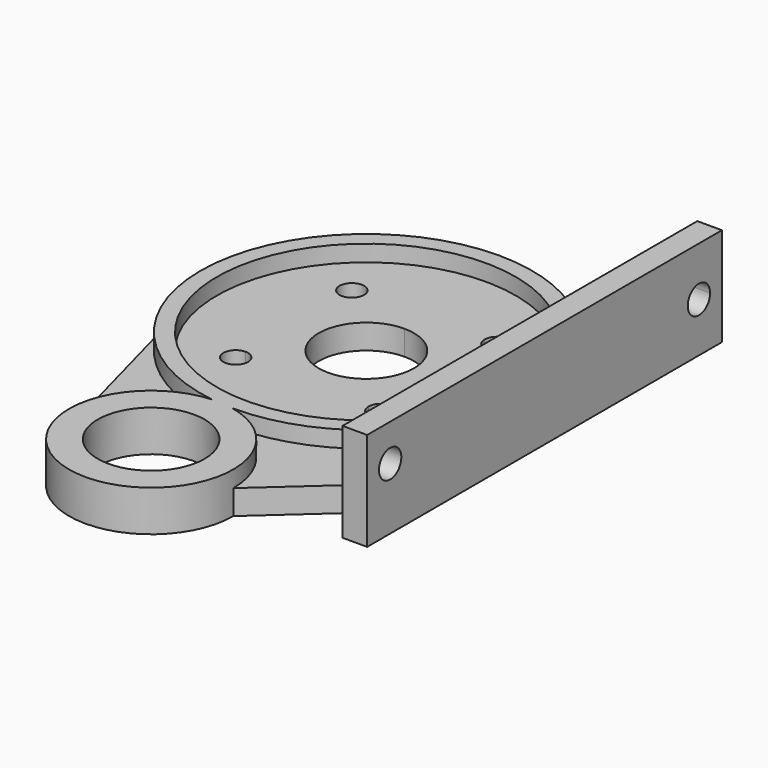
from build123d import *

# Parameters (mm, degrees)
F0_W     = 3
F0_H     = 6.8
F1_DEPTH = 12
F2_DEPTH = 5
F3_DEPTH = 3
F0_R     = 6.5
F4_DEPTH = 5
F5_DEPTH = 3
F7_DEPTH = 25
F8_DEPTH = 25
F9_DEPTH = 3


with BuildPart() as f1:
    # F0 (on Top) → F1 (new body)
    with BuildSketch(Plane.XY):
        with Locations((20.2, 23.6)):
            Rectangle(F0_W, F0_H)
        with BuildLine():
            Line((18.7, 20.2), (18.7, 7.6387171698))
            ThreePointArc((18.7, 7.6387171698), (19.8214530244, 3.8923000912), (20.2, 0))
            Line((20.2, 0), (21.7, 0))
            Line((21.7, 0), (21.7, 20.2))
            Line((21.7, 20.2), (18.7, 20.2))
        make_face()
        with BuildLine():
            Line((21.7, 0), (20.2, 0))
            ThreePointArc((20.2, 0), (19.8214530244, -3.8923000912), (18.7, -7.6387171698))
            Line((18.7, -7.6387171698), (18.7, -20.2))
            Line((18.7, -20.2), (21.7, -20.2))
            Line((21.7, -20.2), (21.7, 0))
        make_face()
        with Locations((20.2, -23.6)):
            Rectangle(F0_W, F0_H)
        with BuildLine():
            ThreePointArc((20.2, 0), (19.8214530244, 3.8923000912), (18.7, 7.6387171698))
            Line((18.7, 7.6387171698), (18.7, 0))
            Line((18.7, 0), (20.2, 0))
        make_face()
        with BuildLine():
            ThreePointArc((18.7, -7.6387171698), (19.8214530244, -3.8923000912), (20.2, 0))
            Line((20.2, 0), (18.7, 0))
            Line((18.7, 0), (18.7, -7.6387171698))
        make_face()
    extrude(amount=F1_DEPTH)

    # F0 (on Top) → F2 (join)
    with BuildSketch(Plane.XY):
        with BuildLine():
            Line((0, 18.2), (0, 20.2))
            ThreePointArc((0, 20.2), (-14.28355698, 14.28355698), (-20.2, 0))
            Line((-20.2, 0), (-17.4867563263, -10.1120400111))
            ThreePointArc((-17.4867563263, -10.1120400111), (-11.2572434768, -16.7724318244), (-2.7332534209, -20.0142280825))
            ThreePointArc((-2.7332534209, -20.0142280825), (-1.4686306009, -20.0267809208), (-0.215705511, -20.1988482625))
            ThreePointArc((-0.215705511, -20.1988482625), (-0.1078542929, -20.1997120636), (0, -20.2))
            Line((0, -20.2), (0, -18.2))
            ThreePointArc((0, -18.2), (-18.2, 0), (0, 18.2))
        make_face()
        with BuildLine():
            ThreePointArc((18.7, 7.6387171698), (11.2636120576, 16.7681556355), (0, 20.2))
            Line((0, 20.2), (0, 18.2))
            ThreePointArc((0, 18.2), (12.8693434176, 12.8693434176), (18.2, 0))
            ThreePointArc((18.2, 0), (12.8693434176, -12.8693434176), (0, -18.2))
            Line((0, -18.2), (0, -20.2))
            ThreePointArc((0, -20.2), (11.2636120576, -16.7681556355), (18.7, -7.6387171698))
            Line((18.7, -7.6387171698), (18.7, 0))
            Line((18.7, 0), (18.7, 7.6387171698))
        make_face()
        with BuildLine():
            Line((-17.4867563263, -10.1120400111), (-20.2, 0))
            ThreePointArc((-20.2, 0), (-19.5099010478, -5.23486018), (-17.4867563263, -10.1120400111))
        make_face()
    extrude(amount=F2_DEPTH)

    # F0 (on Top) → F3 (join)
    with BuildSketch(Plane.XY):
        with BuildLine():
            Line((0, 8.8388347648), (0, 18.2))
            ThreePointArc((0, 18.2), (-18.2, 0), (0, -18.2))
            Line((0, -18.2), (0, -8.8388347648))
            Line((0, -8.8388347648), (-7.3388347648, -8.8388347648))
            ThreePointArc((-7.3388347648, -8.8388347648), (-9.8994949366, -9.8994949366), (-8.8388347648, -7.3388347648))
            Line((-8.8388347648, -7.3388347648), (-8.8388347648, 7.3388347648))
            ThreePointArc((-8.8388347648, 7.3388347648), (-9.8994949366, 9.8994949366), (-7.3388347648, 8.8388347648))
            Line((-7.3388347648, 8.8388347648), (0, 8.8388347648))
        make_face()
        with BuildLine():
            Line((7.3388347648, 8.8388347648), (0, 8.8388347648))
            Line((0, 8.8388347648), (0, 5.8))
            ThreePointArc((0, 5.8), (4.1012193309, 4.1012193309), (5.8, 0))
            ThreePointArc((5.8, 0), (4.1012193309, -4.1012193309), (0, -5.8))
            Line((0, -5.8), (0, -8.8388347648))
            Line((0, -8.8388347648), (7.3388347648, -8.8388347648))
            ThreePointArc((7.3388347648, -8.8388347648), (7.7781745931, -7.7781745931), (8.8388347648, -7.3388347648))
            Line((8.8388347648, -7.3388347648), (8.8388347648, 7.3388347648))
            ThreePointArc((8.8388347648, 7.3388347648), (7.7781745931, 7.7781745931), (7.3388347648, 8.8388347648))
        make_face()
        with BuildLine():
            Line((0, 5.8), (0, 8.8388347648))
            Line((0, 8.8388347648), (-7.3388347648, 8.8388347648))
            ThreePointArc((-7.3388347648, 8.8388347648), (-7.7781745931, 7.7781745931), (-8.8388347648, 7.3388347648))
            Line((-8.8388347648, 7.3388347648), (-8.8388347648, -7.3388347648))
            ThreePointArc((-8.8388347648, -7.3388347648), (-7.7781745931, -7.7781745931), (-7.3388347648, -8.8388347648))
            Line((-7.3388347648, -8.8388347648), (0, -8.8388347648))
            Line((0, -8.8388347648), (0, -5.8))
            ThreePointArc((0, -5.8), (-5.8, 0), (0, 5.8))
        make_face()
        with BuildLine():
            ThreePointArc((18.2, 0), (12.8693434176, 12.8693434176), (0, 18.2))
            Line((0, 18.2), (0, 8.8388347648))
            Line((0, 8.8388347648), (7.3388347648, 8.8388347648))
            ThreePointArc((7.3388347648, 8.8388347648), (8.8388347648, 10.3388347648), (10.3388347648, 8.8388347648))
            ThreePointArc((10.3388347648, 8.8388347648), (9.8994949366, 7.7781745931), (8.8388347648, 7.3388347648))
            Line((8.8388347648, 7.3388347648), (8.8388347648, -7.3388347648))
            ThreePointArc((8.8388347648, -7.3388347648), (9.8994949366, -7.7781745931), (10.3388347648, -8.8388347648))
            ThreePointArc((10.3388347648, -8.8388347648), (8.8388347648, -10.3388347648), (7.3388347648, -8.8388347648))
            Line((7.3388347648, -8.8388347648), (0, -8.8388347648))
            Line((0, -8.8388347648), (0, -18.2))
            ThreePointArc((0, -18.2), (12.8693434176, -12.8693434176), (18.2, 0))
        make_face()
    extrude(amount=F3_DEPTH)

    # F0 (on Top) → F4 (join)
    with BuildSketch(Plane.XY):
        with BuildLine():
            ThreePointArc((-0.215705511, -20.1988482625), (-1.4686306009, -20.0267809208), (-2.7332534209, -20.0142280825))
            ThreePointArc((-2.7332534209, -20.0142280825), (-1.4773661863, -20.14590254), (-0.215705511, -20.1988482625))
        make_face()
        with BuildLine():
            ThreePointArc((-0.215705511, -20.1988482625), (-1.4773661863, -20.14590254), (-2.7332534209, -20.0142280825))
            ThreePointArc((-2.7332534209, -20.0142280825), (-9.3953899149, -23.0554795722), (-12.1984032717, -29.8213046815))
            ThreePointArc((-12.1984032717, -29.8213046815), (-2.2893512261, -39.99960081), (7.8, -30))
            ThreePointArc((7.8, -30), (5.5408961009, -23.6692395753), (-0.215705511, -20.1988482625))
        make_face()
        with Locations((-2.2, -30)):
            Circle(F0_R, mode=Mode.SUBTRACT)
    extrude(amount=F4_DEPTH)

    # F0 (on Top) → F5 (join)
    with BuildSketch(Plane.XY):
        with BuildLine():
            ThreePointArc((-2.7332534209, -20.0142280825), (-11.2572434768, -16.7724318244), (-17.4867563263, -10.1120400111))
            Line((-17.4867563263, -10.1120400111), (-12.1984032717, -29.8213046815))
            ThreePointArc((-12.1984032717, -29.8213046815), (-9.3953899149, -23.0554795722), (-2.7332534209, -20.0142280825))
        make_face()
        with BuildLine():
            Line((18.7, -20.2), (18.7, -7.6387171698))
            ThreePointArc((18.7, -7.6387171698), (11.2636120576, -16.7681556355), (0, -20.2))
            Line((0, -20.2), (18.7, -20.2))
        make_face()
        with BuildLine():
            Line((18.7, -20.2), (0, -20.2))
            ThreePointArc((0, -20.2), (-0.1078542929, -20.1997120636), (-0.215705511, -20.1988482625))
            ThreePointArc((-0.215705511, -20.1988482625), (5.5408961009, -23.6692395753), (7.8, -30))
            Line((7.8, -30), (18.7, -20.2))
        make_face()
    extrude(amount=F5_DEPTH)

    # F6 (on face) → F7 (cut)
    with BuildSketch(Plane(origin=(18.7, 0, 0), x_dir=(0, -1, 0), z_dir=(-1, 0, 0))):
        with BuildLine():
            Line((-25.2, 6), (-23.5, 6))
            Line((-23.5, 6), (-23.5, 7.7))
            ThreePointArc((-23.5, 7.7), (-24.702081528, 7.202081528), (-25.2, 6))
        make_face()
        with BuildLine():
            Line((-21.8, 6), (-23.5, 6))
            Line((-23.5, 6), (-25.2, 6))
            ThreePointArc((-25.2, 6), (-23.5, 4.3), (-21.8, 6))
        make_face()
        with BuildLine():
            Line((-23.5, 7.7), (-23.5, 6))
            Line((-23.5, 6), (-21.8, 6))
            ThreePointArc((-21.8, 6), (-22.297918472, 7.202081528), (-23.5, 7.7))
        make_face()
    extrude(amount=-F7_DEPTH, mode=Mode.SUBTRACT)

    # F6 (on face) → F8 (cut)
    with BuildSketch(Plane(origin=(18.7, 0, 0), x_dir=(0, -1, 0), z_dir=(-1, 0, 0))):
        with BuildLine():
            Line((-21.8, 6), (-23.5, 6))
            Line((-23.5, 6), (-25.2, 6))
            ThreePointArc((-25.2, 6), (-23.5, 4.3), (-21.8, 6))
        make_face()
        with BuildLine():
            Line((-25.2, 6), (-23.5, 6))
            Line((-23.5, 6), (-23.5, 7.7))
            ThreePointArc((-23.5, 7.7), (-24.702081528, 7.202081528), (-25.2, 6))
        make_face()
        with BuildLine():
            Line((-23.5, 7.7), (-23.5, 6))
            Line((-23.5, 6), (-21.8, 6))
            ThreePointArc((-21.8, 6), (-22.297918472, 7.202081528), (-23.5, 7.7))
        make_face()
        with BuildLine():
            ThreePointArc((23.5, 9.2), (22.297918472, 6.297918472), (25.2, 7.5))
            ThreePointArc((25.2, 7.5), (24.702081528, 8.702081528), (23.5, 9.2))
        make_face()
    extrude(amount=-F8_DEPTH, mode=Mode.SUBTRACT)

    # F0 (on Top) → F9 (join)
    with BuildSketch(Plane.XY):
        with BuildLine():
            Line((18.7, 20.2), (0, 20.2))
            ThreePointArc((0, 20.2), (11.2636120576, 16.7681556355), (18.7, 7.6387171698))
            Line((18.7, 7.6387171698), (18.7, 20.2))
        make_face()
    extrude(amount=F9_DEPTH)


with BuildPart() as f10_1:
    # F10: copy of F1
    add(f1.part)


solid = f10_1.part
